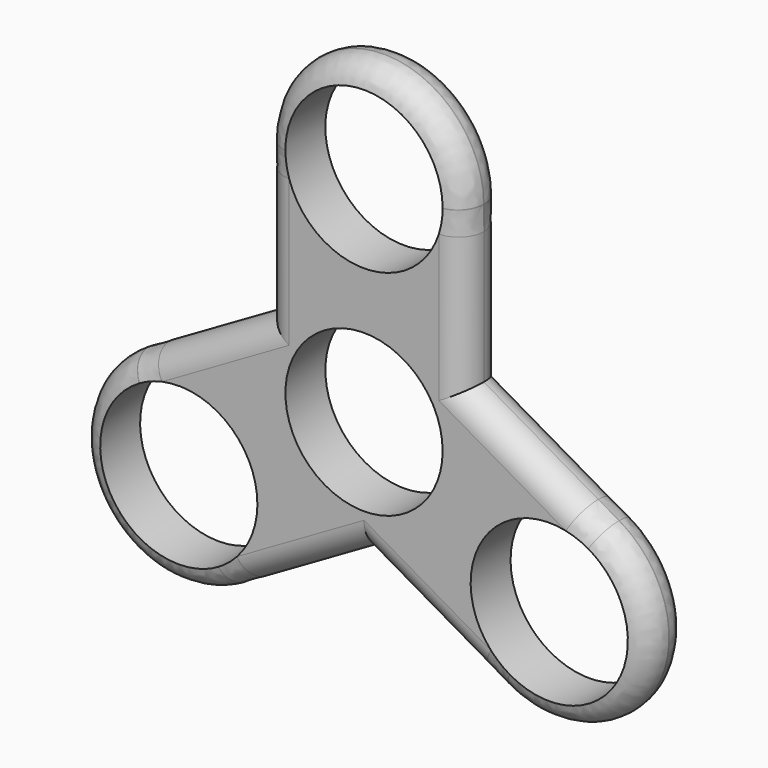
from build123d import *

# Parameters (mm, degrees)
F1_DEPTH = 7
F2_COUNT = 3
F3_R     = 3.49999
F4_R     = 3.5


# Not quite as in the source:
# - a fillet or chamfer is up to 0.001 mm smaller than in the source, because OpenCascade refuses the exact size


with BuildPart() as f1:
    # F0 (on Front) → F1 (new body)
    with BuildSketch(Plane.XZ):
        with BuildLine():
            Line((11.025, 15), (14, 15))
            ThreePointArc((14, 15), (0, 29), (-14, 15))
            Line((-14, 15), (-11.025, 15))
            ThreePointArc((-11.025, 15), (0, 26.025), (11.025, 15))
        make_face()
        with BuildLine():
            ThreePointArc((-14, 15), (0, 1), (14, 15))
            Line((14, 15), (11.025, 15))
            ThreePointArc((11.025, 15), (0, 3.975), (-11.025, 15))
            Line((-11.025, 15), (-14, 15))
        make_face()
        with BuildLine():
            Line((11.025, -15), (14, -15))
            ThreePointArc((14, -15), (0, -1), (-14, -15))
            Line((-14, -15), (-11.025, -15))
            ThreePointArc((-11.025, -15), (0, -3.975), (11.025, -15))
        make_face()
        with BuildLine():
            ThreePointArc((-14, -15), (0, -29), (14, -15))
            Line((14, -15), (11.025, -15))
            ThreePointArc((11.025, -15), (0, -26.025), (-11.025, -15))
            Line((-11.025, -15), (-14, -15))
        make_face()
        with BuildLine():
            ThreePointArc((-14, -15), (0, -1), (14, -15))
            Line((14, -15), (14, 15))
            ThreePointArc((14, 15), (0, 1), (-14, 15))
            Line((-14, 15), (-14, -15))
        make_face()
    extrude(amount=F1_DEPTH)

    # F2: F1 ×3 about axis
    f2_axis = Axis((0, -7, -15), (0, 1, 0))


with BuildPart() as f1_1:
    add(f1.part)
    for i in range(1, F2_COUNT):
        add(f1.part.rotate(f2_axis, i * 360 / F2_COUNT))

    # F3 (radius 3.5 in the source; OpenCascade refuses exactly that, so slightly less here)
    f3_edges = [f1_1.edges().sort_by_distance(p)[0] for p in [
        (0, -7, 29),
        (-14, -7, 4.041452),
        (14, -7, 4.041452),
        (38.105118, -7, -37),
        (9.490381, -7, -36.645082),
        (23.490381, -7, -12.39637),
        (-23.490381, 0, -12.39637),
        (-38.105118, -7, -37),
        (-9.490381, -7, -36.645082),
    ]]
    fillet(f3_edges, radius=F3_R)

    # F4
    f4_edges = [f1_1.edges().sort_by_distance(p)[0] for p in [
        (14, 0, 4.041452),
        (0, 0, 29),
        (9.490381, 0, -36.645082),
        (-14, 0, 4.041452),
        (38.105118, 0, -37),
        (23.490381, 0, -12.39637),
    ]]
    fillet(f4_edges, radius=F4_R)


solid = f1_1.part
